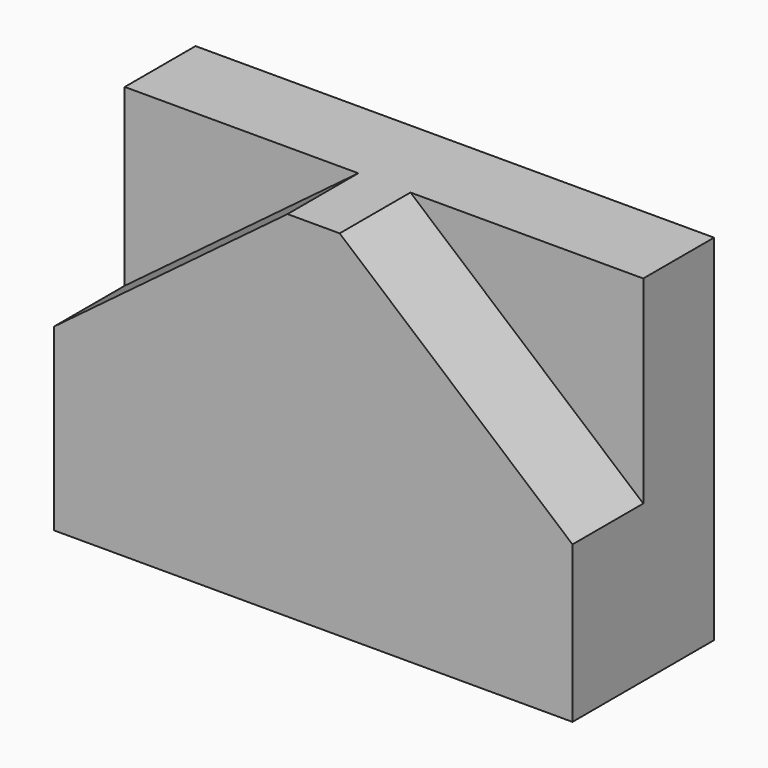
from build123d import *

# Parameters (mm, degrees)
F0_W     = 148.8501727581
F0_H     = 101.742612198
F1_DEPTH = 50.8
F3_DEPTH = 25.4


with BuildPart() as f1:
    # F0 (on Front) → F1 (new body)
    with BuildSketch(Plane.XZ):
        with Locations((-1.6997531056, 25.3749480471)):
            Rectangle(F0_W, F0_H)
    extrude(amount=F1_DEPTH)

    # F2 (on face) → F3 (cut)
    with BuildSketch(Plane.XZ.offset(50.8)):
        Polygon((-9.0788973585, 76.2462541461), (-76.1248394847, 76.2462541461), (-76.1248394847, 26.0104050889), align=None)
        Polygon((72.7253332734, 76.2462541461), (5.8954056378, 76.2462541461), (72.7253332734, 19.3677039224), align=None)
    extrude(amount=-F3_DEPTH, mode=Mode.SUBTRACT)


solid = f1.part
